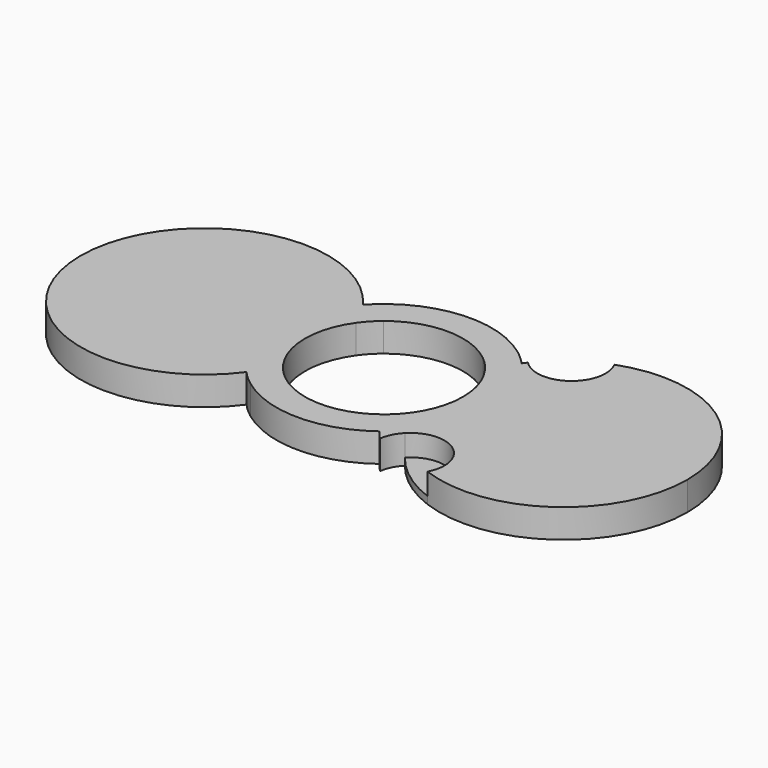
from build123d import *

# Parameters (mm, degrees)
F1_DEPTH = 4
F2_DEPTH = 1


# Not quite as in the source:
# - a feature names something its author has since deleted; it is built from what else it names


with BuildPart() as f1:
    # F0 (on Top) → F1 (new body)
    with BuildSketch(Plane.XY):
        with BuildLine():
            ThreePointArc((33.96875, 44.5973311111), (35.4798914594, 41.5709736662), (36, 38.228538177))
            ThreePointArc((36, 38.228538177), (35.4798914594, 34.8861026877), (33.96875, 31.8597452428))
            ThreePointArc((33.96875, 31.8597452428), (34.890304672, 29.9063024739), (36.04875, 28.083336186))
            ThreePointArc((36.04875, 28.083336186), (38.9773253879, 32.7847917648), (40, 38.228538177))
            ThreePointArc((40, 38.228538177), (38.9773253879, 43.6722845891), (36.04875, 48.3737401679))
            ThreePointArc((36.04875, 48.3737401679), (34.890304672, 46.55077388), (33.96875, 44.5973311111))
        make_face()
        with BuildLine():
            ThreePointArc((31.92, 46.7791872751), (33.0189287452, 45.7582647177), (33.96875, 44.5973311111))
            ThreePointArc((33.96875, 44.5973311111), (34.890304672, 46.55077388), (36.04875, 48.3737401679))
            ThreePointArc((36.04875, 48.3737401679), (35.0671824784, 49.3484229311), (34, 50.228538177))
            ThreePointArc((34, 50.228538177), (32.8729423014, 48.5563595633), (31.92, 46.7791872751))
        make_face()
        with BuildLine():
            ThreePointArc((36.04875, 28.083336186), (34.890304672, 29.9063024739), (33.96875, 31.8597452428))
            ThreePointArc((33.96875, 31.8597452428), (33.0189287452, 30.6988116362), (31.92, 29.6778890788))
            ThreePointArc((31.92, 29.6778890788), (32.8729423014, 27.9007167906), (34, 26.228538177))
            ThreePointArc((34, 26.228538177), (35.0671824784, 27.1086534228), (36.04875, 28.083336186))
        make_face()
        with BuildLine():
            ThreePointArc((18.08, 46.7791872751), (25, 49.228538177), (31.92, 46.7791872751))
            ThreePointArc((31.92, 46.7791872751), (32.8729423014, 48.5563595633), (34, 50.228538177))
            ThreePointArc((34, 50.228538177), (25, 53.228538177), (16, 50.228538177))
            ThreePointArc((16, 50.228538177), (17.1270576986, 48.5563595633), (18.08, 46.7791872751))
        make_face()
        with BuildLine():
            ThreePointArc((36.4851682331, 48.9482313775), (36.2639553749, 48.6632675964), (36.04875, 48.3737401679))
            ThreePointArc((36.04875, 48.3737401679), (38.9773253879, 43.6722845891), (40, 38.228538177))
            ThreePointArc((40, 38.228538177), (38.9773253879, 32.7847917648), (36.04875, 28.083336186))
            ThreePointArc((36.04875, 28.083336186), (36.2190453875, 27.853192883), (36.3931368718, 27.6259075689))
            ThreePointArc((36.3931368718, 27.6259075689), (41.5858805009, 28.7167510128), (44.5495147975, 24.3154560246))
            ThreePointArc((44.5495147975, 24.3154560246), (44.4052654508, 23.1537499865), (43.9812786211, 22.062601985))
            ThreePointArc((43.9812786211, 22.062601985), (59.8422445665, 24.0619323063), (67.25, 38.228538177))
            ThreePointArc((67.25, 38.228538177), (59.9032981891, 52.3525314146), (44.1210510171, 54.4458270643))
            ThreePointArc((44.1210510171, 54.4458270643), (44.5307176941, 53.3709710002), (44.6699958357, 52.2291549274))
            ThreePointArc((44.6699958357, 52.2291549274), (41.6873482182, 47.8201907003), (36.4851682331, 48.9482313775))
        make_face()
        with BuildLine():
            ThreePointArc((50, 45.978538177), (55.4800775542, 43.7086157311), (57.75, 38.228538177))
            ThreePointArc((57.75, 38.228538177), (44.5199224458, 32.7484606228), (50, 45.978538177))
        make_face(mode=Mode.SUBTRACT)
        with BuildLine():
            ThreePointArc((34, 26.228538177), (32.8729423014, 27.9007167906), (31.92, 29.6778890788))
            ThreePointArc((31.92, 29.6778890788), (25, 27.228538177), (18.08, 29.6778890788))
            ThreePointArc((18.08, 29.6778890788), (17.1270576986, 27.9007167906), (16, 26.228538177))
            ThreePointArc((16, 26.228538177), (25, 23.228538177), (34, 26.228538177))
        make_face()
        with BuildLine():
            ThreePointArc((36.3931368718, 27.6259075689), (36.2190453875, 27.853192883), (36.04875, 28.083336186))
            ThreePointArc((36.04875, 28.083336186), (35.0671824784, 27.1086534228), (34, 26.228538177))
            ThreePointArc((34, 26.228538177), (34.528786958, 25.5540927449), (35.0859826327, 24.9029205189))
            ThreePointArc((35.0859826327, 24.9029205189), (35.517354176, 26.3710825501), (36.3931368718, 27.6259075689))
        make_face()
        with BuildLine():
            ThreePointArc((16.03125, 44.5973311111), (16.9810712548, 45.7582647177), (18.08, 46.7791872751))
            ThreePointArc((18.08, 46.7791872751), (17.1270576986, 48.5563595633), (16, 50.228538177))
            ThreePointArc((16, 50.228538177), (14.9328175216, 49.3484229311), (13.95125, 48.3737401679))
            ThreePointArc((13.95125, 48.3737401679), (15.109695328, 46.55077388), (16.03125, 44.5973311111))
        make_face()
        with BuildLine():
            ThreePointArc((16, 26.228538177), (17.1270576986, 27.9007167906), (18.08, 29.6778890788))
            ThreePointArc((18.08, 29.6778890788), (16.9810712548, 30.6988116362), (16.03125, 31.8597452428))
            ThreePointArc((16.03125, 31.8597452428), (15.109695328, 29.9063024739), (13.95125, 28.083336186))
            ThreePointArc((13.95125, 28.083336186), (14.9328175216, 27.1086534228), (16, 26.228538177))
        make_face()
        with BuildLine():
            ThreePointArc((16.03125, 31.8597452428), (14, 38.228538177), (16.03125, 44.5973311111))
            ThreePointArc((16.03125, 44.5973311111), (15.109695328, 46.55077388), (13.95125, 48.3737401679))
            ThreePointArc((13.95125, 48.3737401679), (10, 38.228538177), (13.95125, 28.083336186))
            ThreePointArc((13.95125, 28.083336186), (15.109695328, 29.9063024739), (16.03125, 31.8597452428))
        make_face()
        with BuildLine():
            ThreePointArc((13.95125, 28.083336186), (10, 38.228538177), (13.95125, 48.3737401679))
            ThreePointArc((13.95125, 48.3737401679), (-17.25, 38.228538177), (13.95125, 28.083336186))
        make_face()
        with BuildLine():
            ThreePointArc((0, 45.978538177), (5.4800775542, 43.7086157311), (7.75, 38.228538177))
            ThreePointArc((7.75, 38.228538177), (-5.4800775542, 32.7484606228), (0, 45.978538177))
        make_face(mode=Mode.SUBTRACT)
        with BuildLine():
            ThreePointArc((0, 45.978538177), (-5.4800775542, 32.7484606228), (7.75, 38.228538177))
            ThreePointArc((7.75, 38.228538177), (5.4800775542, 43.7086157311), (0, 45.978538177))
        make_face()
        with BuildLine():
            ThreePointArc((50, 45.978538177), (44.5199224458, 32.7484606228), (57.75, 38.228538177))
            ThreePointArc((57.75, 38.228538177), (55.4800775542, 43.7086157311), (50, 45.978538177))
        make_face()
    extrude(amount=F1_DEPTH)

    # F0 (on Top) → F2 (join)
    with BuildSketch(Plane.XY):
        with BuildLine():
            ThreePointArc((44.1210510171, 54.4458270643), (39.9210331617, 52.2277141339), (36.4851682331, 48.9482313775))
            ThreePointArc((36.4851682331, 48.9482313775), (41.6873482182, 47.8201907003), (44.6699958357, 52.2291549274))
            ThreePointArc((44.6699958357, 52.2291549274), (44.5307176941, 53.3709710002), (44.1210510171, 54.4458270643))
        make_face()
        with BuildLine():
            ThreePointArc((44.5495147975, 24.3154560246), (41.5858805009, 28.7167510128), (36.3931368718, 27.6259075689))
            ThreePointArc((36.3931368718, 27.6259075689), (39.8005645222, 24.31688781), (43.9812786211, 22.062601985))
            ThreePointArc((43.9812786211, 22.062601985), (44.4052654508, 23.1537499865), (44.5495147975, 24.3154560246))
        make_face()
    extrude(amount=F2_DEPTH)


solid = f1.part
